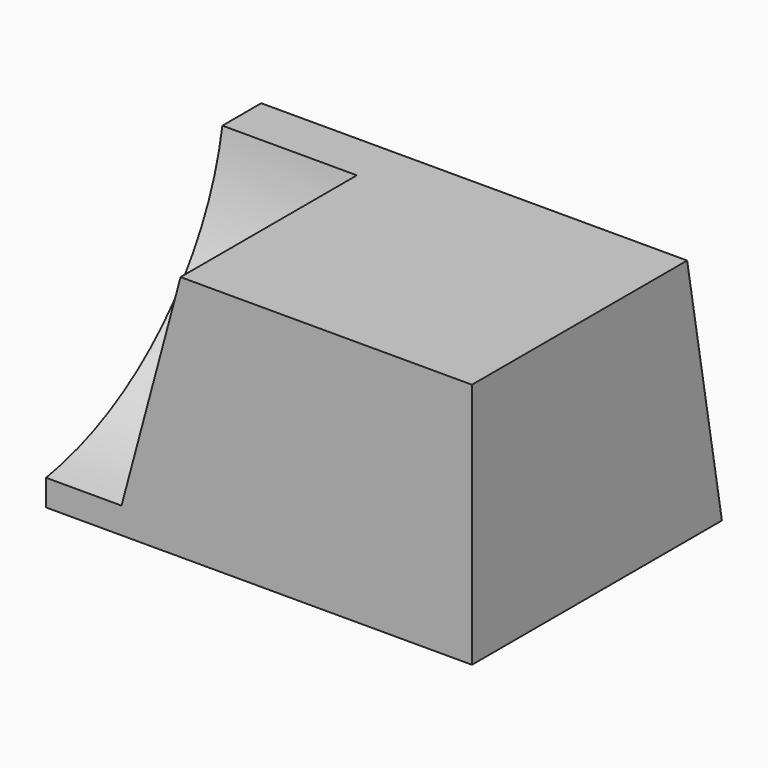
from build123d import *

# Parameters (mm, degrees)
F0_W     = 190
F0_H     = 120
F1_DEPTH = 110
F3_DEPTH = 190
F7_REACH = 199.0477340594


with BuildPart() as f1:
    # F0 (on Top) → F1 (new body)
    with BuildSketch(Plane.XY):
        Rectangle(F0_W, F0_H)
    extrude(amount=-F1_DEPTH)

    # F2 (on face) → F3 (join, through all)
    with BuildSketch(Plane.YZ.offset(95)):
        Polygon((79.3959678779, -110), (60, 0), (60, -110), align=None)
    extrude(amount=-F3_DEPTH)

    f7_end = Plane(origin=(-32.6554445662, 0, 8.75), x_dir=(0.2588190451, 0, 0.9659258263), z_dir=(0.9659258263, 0, -0.2588190451))
    # F4 (on face) → F7 (cut, up to a plane its end follows)
    with BuildSketch(Plane(origin=(-95, 0, 0), x_dir=(0, -1, 0), z_dir=(-1, 0, 0))):
        with BuildLine():
            Line((60, -98.321595662), (60, 0))
            Line((60, 0), (-38.321595662, 0))
            ThreePointArc((-38.321595662, 0), (-4.8528137424, -64.8528137424), (60, -98.321595662))
        make_face()
    f7_long = extrude(amount=-F7_REACH, mode=Mode.PRIVATE)
    add(split(f7_long, bisect_by=f7_end, keep=Keep.BOTTOM, mode=Mode.PRIVATE), mode=Mode.SUBTRACT)


solid = f1.part
